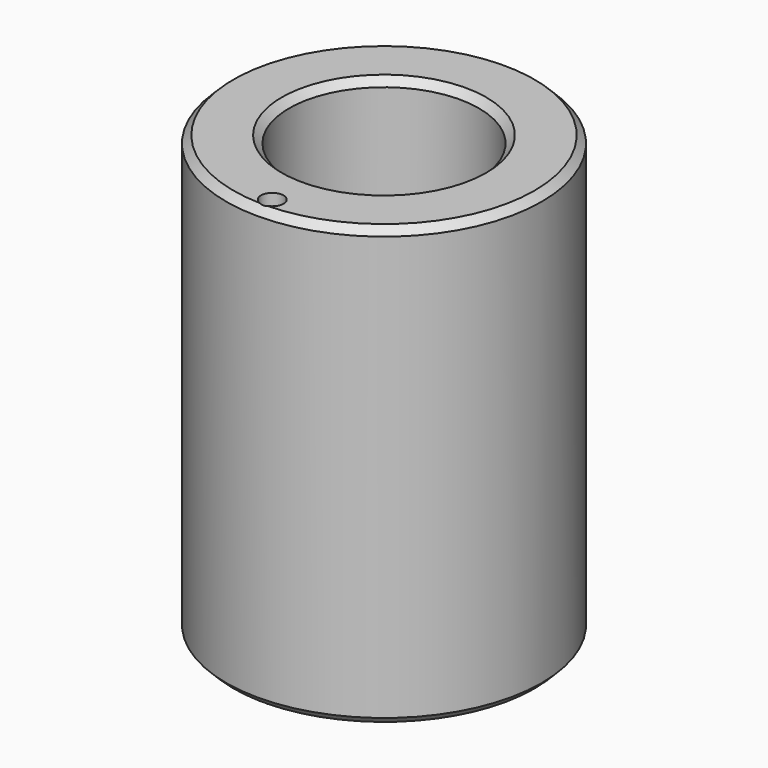
from build123d import *

# Parameters (mm, degrees)
F0_R     = 5.4
F0_R_2   = 0.3873329086
F0_R_3   = 3.25
F1_DEPTH = 15


# Not quite as in the source:
# - a fillet or chamfer that OpenCascade refuses, or shapes differently, is made with other operations: its cross-section is extruded or revolved along the edge and cut away or added


with BuildPart() as f1:
    # F0 (on Top) → F1 (new body)
    with BuildSketch(Plane.XY):
        Circle(F0_R)
        with Locations((0, -4.7800762477)):
            Circle(F0_R_2, mode=Mode.SUBTRACT)
        Circle(F0_R_3, mode=Mode.SUBTRACT)
    extrude(amount=F1_DEPTH)

    # F2: chamfer of 0.25 on 3 edges, made by hand

    # F2_s1 → F2_t2 (revolve, cut)
    with BuildSketch(Plane.XZ):
        Polygon((3.25, 14.75), (3.5, 15), (3.25, 15), align=None)
    revolve(axis=Axis((0, 0, 15), (0, 0, 1)), mode=Mode.SUBTRACT)

    # F2_s3 → F2_t4 (revolve, cut)
    with BuildSketch(Plane.XZ):
        Polygon((5.4, 14.75), (5.15, 15), (5.4, 15), align=None)
    revolve(axis=Axis((0, 0, 15), (0, 0, 1)), mode=Mode.SUBTRACT)

    # F2_s5 → F2_t6 (revolve, cut)
    with BuildSketch(Plane.XZ):
        Polygon((3.25, 0.25), (3.5, 0), (3.25, 0), align=None)
    revolve(axis=Axis((0, 0, 0), (0, 0, 1)), mode=Mode.SUBTRACT)

    # F3: chamfer of 0.25 on 1 edges, made by hand

    # F3_s1 → F3_t2 (revolve, cut)
    with BuildSketch(Plane.XZ):
        Polygon((5.4, 0.25), (5.15, 0), (5.4, 0), align=None)
    revolve(axis=Axis((0, 0, 0), (0, 0, 1)), mode=Mode.SUBTRACT)


solid = f1.part
